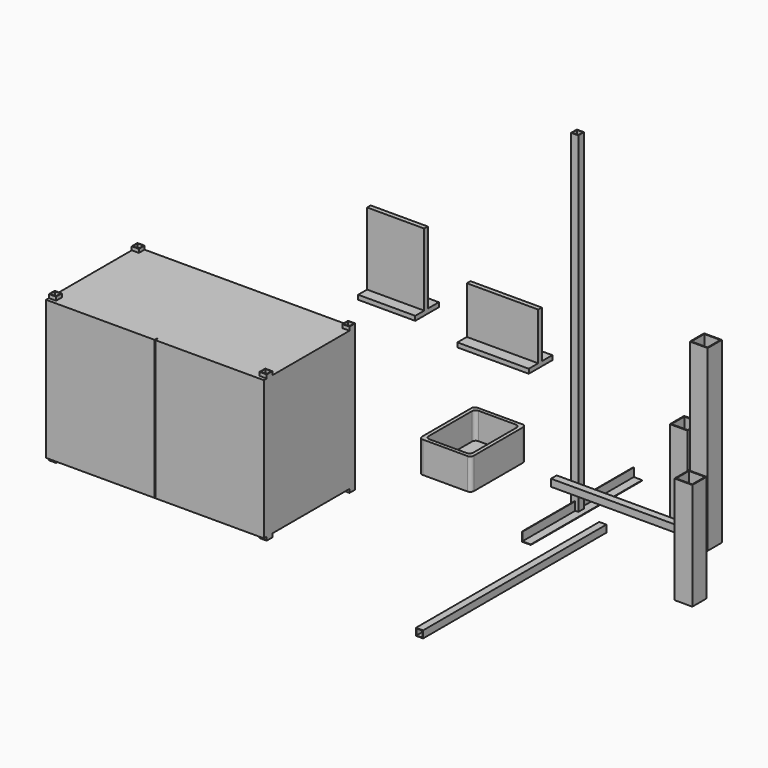
from build123d import *

# Parameters (mm, degrees)
F1_DEPTH  = 390
F2_W      = 40
F2_H      = 40
F2_W_2    = 34
F2_H_2    = 34
F3_DEPTH  = 1860
F4_W      = 40
F4_H      = 40
F4_W_2    = 34
F4_H_2    = 34
F5_DEPTH  = 720
F6_W      = 40
F6_H      = 40
F6_W_2    = 34
F6_H_2    = 34
F7_DEPTH  = 1284
F8_W      = 290
F8_H      = 385
F9_DEPTH  = 25
F10_W     = 290
F10_H     = 385
F10_W_2   = 250
F10_H_2   = 345
F11_DEPTH = 150
F12_R     = 20
F13_W     = 100
F13_H     = 100
F13_W_2   = 90.0000095367
F13_H_2   = 90.0000095367
F14_DEPTH = 505
F15_W     = 100
F15_H     = 100
F15_W_2   = 90
F15_H_2   = 90
F16_DEPTH = 600
F17_W     = 100
F17_H     = 100
F17_W_2   = 90
F17_H_2   = 90
F18_DEPTH = 1000
F19_W     = 1220
F19_H     = 620
F20_DEPTH = 780
F21_W     = 40
F21_H     = 40
F21_W_2   = 34
F21_H_2   = 34
F22_DEPTH = 20
F24_DEPTH = 20
F25_W     = 40
F25_H     = 40
F25_W_2   = 34
F25_H_2   = 34
F26_DEPTH = 20
F27_W     = 320
F27_H     = 165
F28_DEPTH = 25
F29_W     = 320
F29_H     = 25
F30_DEPTH = 405
F31_W     = 25
F31_H     = 77.3133778572
F32_DEPTH = 405
F34_DEPTH = 25
F35_W     = 400
F35_H     = 165
F36_DEPTH = 25
F37_W     = 400
F37_H     = 25
F38_DEPTH = 265
F39_W     = 25
F39_H     = 73.8899850845
F40_DEPTH = 264.8
F42_DEPTH = 25
F43_W     = 1140
F43_H     = 749.1722106934
F44_DEPTH = 600


with BuildPart() as f1:
    # F0 (on Front) → F1 (new body, symmetric)
    with BuildSketch(Plane.XZ):
        Polygon((0, 50), (0, 0), (50, 0), (50, 3), (3, 3), (3, 50), align=None)
    extrude(amount=F1_DEPTH, both=True)


with BuildPart() as f3:
    # F2 (on Top) → F3 (new body)
    with BuildSketch(Plane.XY):
        Rectangle(F2_W, F2_H)
        Rectangle(F2_W_2, F2_H_2, mode=Mode.SUBTRACT)
    extrude(amount=F3_DEPTH)


with BuildPart() as f5:
    # F4 (on Right) → F5 (new body)
    with BuildSketch(Plane.YZ):
        with Locations((-165.917519927, 207.9017800093)):
            Rectangle(F4_W, F4_H)
        with Locations((-165.917519927, 207.9017800093)):
            Rectangle(F4_W_2, F4_H_2, mode=Mode.SUBTRACT)
    extrude(amount=F5_DEPTH)


with BuildPart() as f7:
    # F6 (on Front) → F7 (new body)
    with BuildSketch(Plane.XZ):
        with Locations((141.8365803361, -41.3270699978)):
            Rectangle(F6_W, F6_H)
        with Locations((141.8365803361, -41.3270699978)):
            Rectangle(F6_W_2, F6_H_2, mode=Mode.SUBTRACT)
    extrude(amount=F7_DEPTH)


with BuildPart() as f9:
    # F8 (on Top) → F9 (new body)
    with BuildSketch(Plane.XY):
        with Locations((-608.2690548897, 25.2017277479)):
            Rectangle(F8_W, F8_H)
    extrude(amount=F9_DEPTH)

    # F10 (on face) → F11 (join)
    with BuildSketch(Plane.XY.offset(25)):
        with Locations((-608.2690548897, 25.2017277479)):
            Rectangle(F10_W, F10_H)
        with Locations((-608.2690548897, 25.2017277479)):
            Rectangle(F10_W_2, F10_H_2, mode=Mode.SUBTRACT)
    extrude(amount=F11_DEPTH)

    # F12
    f12_edges = [f9.edges().sort_by_distance(p)[0] for p in [
        (-463.269055, -167.298272, 87.5),
        (-463.269055, 217.701728, 87.5),
        (-753.269055, -167.298272, 87.5),
        (-753.269055, 217.701728, 87.5),
        (-733.269055, 197.701728, 100),
        (-483.269055, 197.701728, 100),
        (-483.269055, -147.298272, 100),
        (-733.269055, -147.298272, 100),
    ]]
    fillet(f12_edges, radius=F12_R)


with BuildPart() as f14:
    # F13 (on Top) → F14 (new body)
    with BuildSketch(Plane.XY):
        with Locations((465.7528162003, 176.9267350435)):
            Rectangle(F13_W, F13_H)
        with Locations((465.7528162003, 176.9267350435)):
            Rectangle(F13_W_2, F13_H_2, mode=Mode.SUBTRACT)
    extrude(amount=F14_DEPTH)


with BuildPart() as f16:
    # F15 (on Top) → F16 (new body)
    with BuildSketch(Plane.XY):
        with Locations((917.1401381493, -355.0306677818)):
            Rectangle(F15_W, F15_H)
        with Locations((917.1401381493, -355.0306677818)):
            Rectangle(F15_W_2, F15_H_2, mode=Mode.SUBTRACT)
    extrude(amount=F16_DEPTH)


with BuildPart() as f18:
    # F17 (on Top) → F18 (new body)
    with BuildSketch(Plane.XY):
        with Locations((638.9368057251, 100.0435903668)):
            Rectangle(F17_W, F17_H)
        with Locations((638.9368057251, 100.0435903668)):
            Rectangle(F17_W_2, F17_H_2, mode=Mode.SUBTRACT)
    extrude(amount=F18_DEPTH)


with BuildPart() as f20:
    # F19 (on Top) → F20 (new body)
    with BuildSketch(Plane.XY):
        with Locations((-1511.6287612915, -740.3115653992)):
            Rectangle(F19_W, F19_H)
    extrude(amount=F20_DEPTH)

    # F21 (on face) → F22 (join)
    with BuildSketch(Plane.XY.offset(780)):
        with Locations((-2101.6287612915, -450.3115653992)):
            Rectangle(F21_W, F21_H)
        with Locations((-2101.6287612915, -450.3115653992)):
            Rectangle(F21_W_2, F21_H_2, mode=Mode.SUBTRACT)
        with Locations((-921.6287612915, -450.3115653992)):
            Rectangle(F21_W, F21_H)
        with Locations((-921.6287612915, -450.3115653992)):
            Rectangle(F21_W_2, F21_H_2, mode=Mode.SUBTRACT)
        with Locations((-921.6287612915, -1030.3115653992)):
            Rectangle(F21_W, F21_H)
        with Locations((-921.6287612915, -1030.3115653992)):
            Rectangle(F21_W_2, F21_H_2, mode=Mode.SUBTRACT)
        with Locations((-2101.6287612915, -1030.3115653992)):
            Rectangle(F21_W, F21_H)
        with Locations((-2101.6287612915, -1030.3115653992)):
            Rectangle(F21_W_2, F21_H_2, mode=Mode.SUBTRACT)
    extrude(amount=F22_DEPTH)

    # F23 (on face) → F24 (join)
    with BuildSketch(Plane.XZ.offset(1050.3115653992)):
        Polygon((-941.6287612915, 780), (-1509.6287612915, 780), (-1509.6287612915, 0), (-901.6287612915, 0), (-901.6287612915, 780), align=None)
        Polygon((-1513.6287612915, 0), (-1513.6287612915, 780), (-2081.6287612915, 780), (-2121.6287612915, 780), (-2121.6287612915, 0), align=None)
    extrude(amount=F24_DEPTH)

    # F25 (on face) → F26 (join)
    with BuildSketch(Plane(origin=(0, 0, 0), x_dir=(1, 0, 0), z_dir=(0, 0, -1))):
        with Locations((-921.6287612915, 1030.3115653992)):
            Rectangle(F25_W, F25_H)
        with Locations((-921.6287612915, 1030.3115653992)):
            Rectangle(F25_W_2, F25_H_2, mode=Mode.SUBTRACT)
        with Locations((-2101.6287612915, 1030.3115653992)):
            Rectangle(F25_W, F25_H)
        with Locations((-2101.6287612915, 1030.3115653992)):
            Rectangle(F25_W_2, F25_H_2, mode=Mode.SUBTRACT)
        with Locations((-2101.6287612915, 450.3115653992)):
            Rectangle(F25_W, F25_H)
        with Locations((-2101.6287612915, 450.3115653992)):
            Rectangle(F25_W_2, F25_H_2, mode=Mode.SUBTRACT)
        with Locations((-921.6287612915, 450.3115653992)):
            Rectangle(F25_W, F25_H)
        with Locations((-921.6287612915, 450.3115653992)):
            Rectangle(F25_W_2, F25_H_2, mode=Mode.SUBTRACT)
    extrude(amount=F26_DEPTH)

    # F43 (on face) → F44 (cut)
    with BuildSketch(Plane(origin=(0, -430.3115653992, 0), x_dir=(-1, 0, 0), z_dir=(0, 1, 0))):
        with Locations((1511.6287612915, 374.5861053467)):
            Rectangle(F43_W, F43_H)
    extrude(amount=-F44_DEPTH, mode=Mode.SUBTRACT)


with BuildPart() as f28:
    # F27 (on Top) → F28 (new body)
    with BuildSketch(Plane.XY):
        with Locations((-1831.3033914566, 1034.9359107018)):
            Rectangle(F27_W, F27_H)
    extrude(amount=F28_DEPTH)

    # F29 (on face) → F30 (join)
    with BuildSketch(Plane.XY.offset(25)):
        with Locations((-1831.3033914566, 1027.6225328445)):
            Rectangle(F29_W, F29_H)
    extrude(amount=F30_DEPTH)

    # F31 (on face) → F32 (join)
    with BuildSketch(Plane.XY.offset(25)):
        with Locations((-1831.3033914566, 1078.7792217731)):
            Rectangle(F31_W, F31_H)
    extrude(amount=F32_DEPTH)

    # F33 (on face) → F34 (cut)
    with BuildSketch(Plane.YZ.offset(-1818.8033914566)):
        Polygon((1117.4359107018, 430), (1040.1225328445, 430), (1117.4359107018, 25), align=None)
    extrude(amount=-F34_DEPTH, mode=Mode.SUBTRACT)


with BuildPart() as f36:
    # F35 (on Top) → F36 (new body)
    with BuildSketch(Plane.XY):
        with Locations((-1170.1606631279, 953.6658716202)):
            Rectangle(F35_W, F35_H)
    extrude(amount=F36_DEPTH)

    # F37 (on face) → F38 (join)
    with BuildSketch(Plane.XY.offset(25)):
        with Locations((-1170.1606631279, 949.7758865356)):
            Rectangle(F37_W, F37_H)
    extrude(amount=F38_DEPTH)

    # F39 (on face) → F40 (join)
    with BuildSketch(Plane.XY.offset(25)):
        with Locations((-1170.1606631279, 999.2208790779)):
            Rectangle(F39_W, F39_H)
    extrude(amount=F40_DEPTH)

    # F41 (on face) → F42 (cut)
    with BuildSketch(Plane.YZ.offset(-1157.6606631279)):
        Polygon((1036.1658716202, 289.8), (962.2758865356, 289.8), (1036.1658716202, 25), align=None)
    extrude(amount=-F42_DEPTH, mode=Mode.SUBTRACT)


solid = Compound([f1.part, f3.part, f5.part, f7.part, f9.part, f14.part, f16.part, f18.part, f20.part, f28.part, f36.part])
